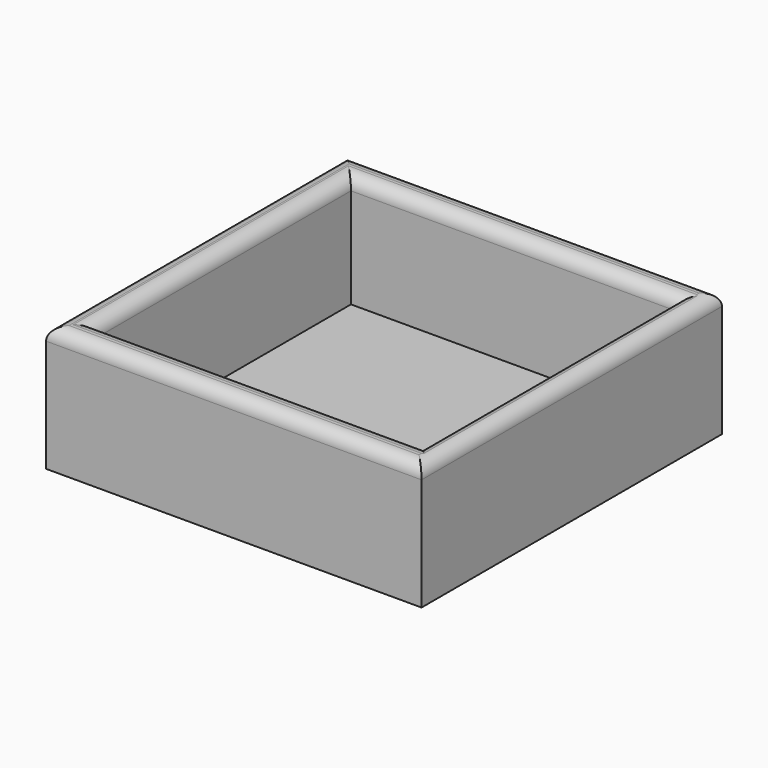
from build123d import *

# Parameters (mm, degrees)
F0_W         = 150
F0_H         = 150
F1_DEPTH     = 50
F2_W         = 130.2189305425
F2_H         = 127.2944062948
F3_DEPTH     = 45
F4_T1_DEPTH  = 175.4
F4_T3_DEPTH  = 175.4
F4_T5_DEPTH  = 127.2944062948
F4_T7_DEPTH  = 130.2189305425
F4_T13_DEPTH = 142.9189305425
F4_T17_DEPTH = 139.9944062948
F4_T24_DEPTH = 139.9944062948
F4_T28_DEPTH = 142.9189305425
F4_T35_DEPTH = 139.9944062948
F4_T39_DEPTH = 142.9189305425
F4_T46_DEPTH = 139.9944062948
F4_T50_DEPTH = 142.9189305425


# Not quite as in the source:
# - a fillet or chamfer that OpenCascade refuses, or shapes differently, is made with other operations: its cross-section is extruded or revolved along the edge and cut away or added


with BuildPart() as f1:
    # F0 (on Top) → F1 (new body)
    with BuildSketch(Plane.XY):
        Rectangle(F0_W, F0_H)
    extrude(amount=F1_DEPTH)

    # F2 (on face) → F3 (cut)
    with BuildSketch(Plane.XY.offset(50)):
        with Locations((0.9621791542, 0.0429600477)):
            Rectangle(F2_W, F2_H)
    extrude(amount=-F3_DEPTH, mode=Mode.SUBTRACT)

    # F4: fillet of radius 5.08 on 8 edges, made by hand

    # F4_s2 → F4_t1 (cut)
    with BuildSketch(Plane.YZ.offset(-87.7)):
        with BuildLine():
            ThreePointArc((69.92, 50), (73.5121024484, 48.5121024484), (75, 44.92))
            Line((75, 44.92), (75, 50))
            Line((75, 50), (69.92, 50))
        make_face()
        with BuildLine():
            ThreePointArc((-75, 44.92), (-73.5121024484, 48.5121024484), (-69.92, 50))
            Line((-69.92, 50), (-75, 50))
            Line((-75, 50), (-75, 44.92))
        make_face()
    extrude(amount=F4_T1_DEPTH, mode=Mode.SUBTRACT)

    # F4_s4 → F4_t3 (cut)
    with BuildSketch(Plane.XZ.offset(-87.7)):
        with BuildLine():
            ThreePointArc((-75, 44.92), (-73.5121024484, 48.5121024484), (-69.92, 50))
            Line((-69.92, 50), (-75, 50))
            Line((-75, 50), (-75, 44.92))
        make_face()
        with BuildLine():
            ThreePointArc((75, 44.92), (73.5121024484, 48.5121024484), (69.92, 50))
            Line((69.92, 50), (75, 50))
            Line((75, 50), (75, 44.92))
        make_face()
    extrude(amount=F4_T3_DEPTH, mode=Mode.SUBTRACT)

    # F4_s6 → F4_t5 (cut)
    with BuildSketch(Plane.XZ.offset(-63.6901631951)):
        with BuildLine():
            ThreePointArc((71.1516444254, 50), (67.559541977, 48.5121024484), (66.0716444254, 44.92))
            Line((66.0716444254, 44.92), (66.0716444254, 50))
            Line((66.0716444254, 50), (71.1516444254, 50))
        make_face()
        with BuildLine():
            ThreePointArc((-69.2272861171, 50), (-65.6351836686, 48.5121024484), (-64.1472861171, 44.92))
            Line((-64.1472861171, 44.92), (-64.1472861171, 50))
            Line((-64.1472861171, 50), (-69.2272861171, 50))
        make_face()
    extrude(amount=F4_T5_DEPTH, mode=Mode.SUBTRACT)

    # F4_s8 → F4_t7 (cut)
    with BuildSketch(Plane.YZ.offset(-64.1472861171)):
        with BuildLine():
            ThreePointArc((-68.6842430997, 50), (-65.0921406513, 48.5121024484), (-63.6042430997, 44.92))
            Line((-63.6042430997, 44.92), (-63.6042430997, 50))
            Line((-63.6042430997, 50), (-68.6842430997, 50))
        make_face()
        with BuildLine():
            ThreePointArc((68.7701631951, 50), (65.1780607467, 48.5121024484), (63.6901631951, 44.92))
            Line((63.6901631951, 44.92), (63.6901631951, 50))
            Line((63.6901631951, 50), (68.7701631951, 50))
        make_face()
    extrude(amount=F4_T7_DEPTH, mode=Mode.SUBTRACT)


with BuildPart() as f4_tool11:
    # F4_s12 → F4_t13 (new body)
    with BuildSketch(Plane.YZ.offset(-64.1472861171)):
        with BuildLine():
            ThreePointArc((-68.6842430997, 50), (-65.0921406513, 48.5121024484), (-63.6042430997, 44.92))
            Line((-63.6042430997, 44.92), (-63.6042430997, 50))
            Line((-63.6042430997, 50), (-68.6842430997, 50))
        make_face()
    extrude(amount=F4_T13_DEPTH)

    split(bisect_by=Plane.YZ.offset(66.0716444254), keep=Keep.TOP)


with BuildPart() as f4_tool15:
    # F4_s16 → F4_t17 (new body)
    with BuildSketch(Plane.XZ.offset(76.3042430997)):
        with BuildLine():
            ThreePointArc((71.1516444254, 50), (67.559541977, 48.5121024484), (66.0716444254, 44.92))
            Line((66.0716444254, 44.92), (66.0716444254, 50))
            Line((66.0716444254, 50), (71.1516444254, 50))
        make_face()
    extrude(amount=-F4_T17_DEPTH)

    split(bisect_by=Plane.XZ.offset(63.6042430997), keep=Keep.TOP)


with BuildPart() as f4_tool11_1:
    add(f4_tool11.part)

    # F4_t19: intersect F4_tool15
    add(f4_tool15.part, mode=Mode.INTERSECT)


with BuildPart() as f1_1:
    add(f1.part)

    # F4_t9: cut F4_tool11
    add(f4_tool11_1.part, mode=Mode.SUBTRACT)


with BuildPart() as f4_tool22:
    # F4_s23 → F4_t24 (new body)
    with BuildSketch(Plane.XZ.offset(63.6042430997)):
        with BuildLine():
            ThreePointArc((71.1516444254, 50), (67.559541977, 48.5121024484), (66.0716444254, 44.92))
            Line((66.0716444254, 44.92), (66.0716444254, 50))
            Line((66.0716444254, 50), (71.1516444254, 50))
        make_face()
    extrude(amount=-F4_T24_DEPTH)

    split(bisect_by=Plane.XZ.offset(-63.6901631951), keep=Keep.BOTTOM)


with BuildPart() as f4_tool26:
    # F4_s27 → F4_t28 (new body)
    with BuildSketch(Plane.YZ.offset(78.7716444254)):
        with BuildLine():
            ThreePointArc((68.7701631951, 50), (65.1780607467, 48.5121024484), (63.6901631951, 44.92))
            Line((63.6901631951, 44.92), (63.6901631951, 50))
            Line((63.6901631951, 50), (68.7701631951, 50))
        make_face()
    extrude(amount=-F4_T28_DEPTH)

    split(bisect_by=Plane.YZ.offset(66.0716444254), keep=Keep.TOP)


with BuildPart() as f4_tool22_1:
    add(f4_tool22.part)

    # F4_t30: intersect F4_tool26
    add(f4_tool26.part, mode=Mode.INTERSECT)


with BuildPart() as f1_2:
    add(f1_1.part)

    # F4_t20: cut F4_tool22
    add(f4_tool22_1.part, mode=Mode.SUBTRACT)


with BuildPart() as f4_tool33:
    # F4_s34 → F4_t35 (new body)
    with BuildSketch(Plane.XZ.offset(-63.6901631951)):
        with BuildLine():
            ThreePointArc((-69.2272861171, 50), (-65.6351836686, 48.5121024484), (-64.1472861171, 44.92))
            Line((-64.1472861171, 44.92), (-64.1472861171, 50))
            Line((-64.1472861171, 50), (-69.2272861171, 50))
        make_face()
    extrude(amount=F4_T35_DEPTH)

    split(bisect_by=Plane.XZ.offset(63.6042430997), keep=Keep.TOP)


with BuildPart() as f4_tool37:
    # F4_s38 → F4_t39 (new body)
    with BuildSketch(Plane.YZ.offset(-76.8472861171)):
        with BuildLine():
            ThreePointArc((-68.6842430997, 50), (-65.0921406513, 48.5121024484), (-63.6042430997, 44.92))
            Line((-63.6042430997, 44.92), (-63.6042430997, 50))
            Line((-63.6042430997, 50), (-68.6842430997, 50))
        make_face()
    extrude(amount=F4_T39_DEPTH)

    split(bisect_by=Plane.YZ.offset(-64.1472861171), keep=Keep.BOTTOM)


with BuildPart() as f4_tool33_1:
    add(f4_tool33.part)

    # F4_t41: intersect F4_tool37
    add(f4_tool37.part, mode=Mode.INTERSECT)


with BuildPart() as f1_3:
    add(f1_2.part)

    # F4_t31: cut F4_tool33
    add(f4_tool33_1.part, mode=Mode.SUBTRACT)


with BuildPart() as f4_tool44:
    # F4_s45 → F4_t46 (new body)
    with BuildSketch(Plane.XZ.offset(-76.3901631951)):
        with BuildLine():
            ThreePointArc((-69.2272861171, 50), (-65.6351836686, 48.5121024484), (-64.1472861171, 44.92))
            Line((-64.1472861171, 44.92), (-64.1472861171, 50))
            Line((-64.1472861171, 50), (-69.2272861171, 50))
        make_face()
    extrude(amount=F4_T46_DEPTH)

    split(bisect_by=Plane.XZ.offset(-63.6901631951), keep=Keep.BOTTOM)


with BuildPart() as f4_tool48:
    # F4_s49 → F4_t50 (new body)
    with BuildSketch(Plane.YZ.offset(66.0716444254)):
        with BuildLine():
            ThreePointArc((68.7701631951, 50), (65.1780607467, 48.5121024484), (63.6901631951, 44.92))
            Line((63.6901631951, 44.92), (63.6901631951, 50))
            Line((63.6901631951, 50), (68.7701631951, 50))
        make_face()
    extrude(amount=-F4_T50_DEPTH)

    split(bisect_by=Plane.YZ.offset(-64.1472861171), keep=Keep.BOTTOM)


with BuildPart() as f4_tool44_1:
    add(f4_tool44.part)

    # F4_t52: intersect F4_tool48
    add(f4_tool48.part, mode=Mode.INTERSECT)


with BuildPart() as f1_4:
    add(f1_3.part)

    # F4_t42: cut F4_tool44
    add(f4_tool44_1.part, mode=Mode.SUBTRACT)


solid = f1_4.part
